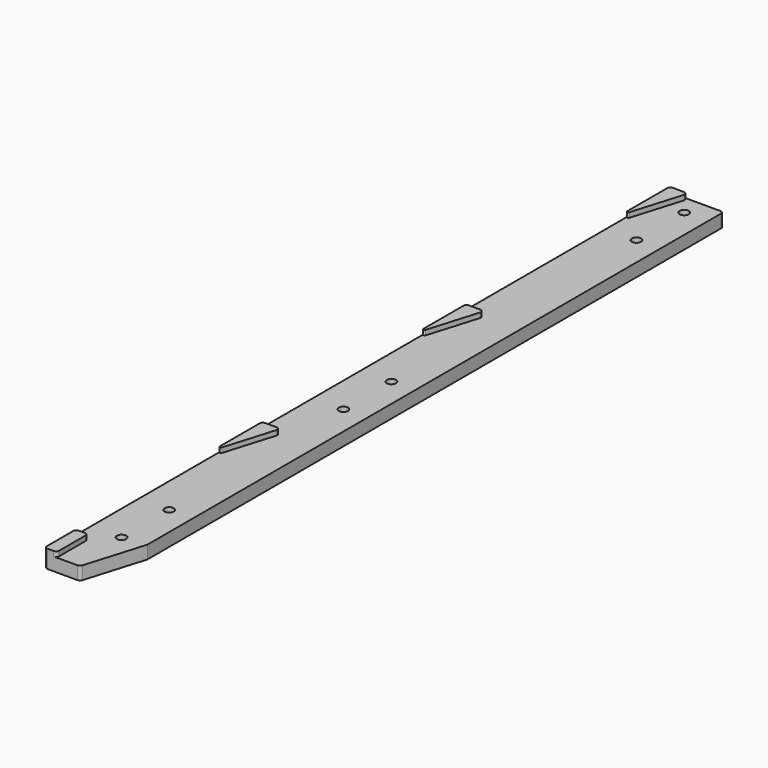
from build123d import *

# Parameters (mm, degrees)
F1_DEPTH = 4.25
F2_W     = 4
F2_H     = 12.7
F3_DEPTH = 1.5875
F4_R     = 1
F5_F1_R  = 0.4
F5_F2_R  = 0.4
F5_F3_R  = 0.4
F7_D     = 3


with BuildPart() as f1:
    # F0 (on Top) → F1 (new body)
    with BuildSketch(Plane.XY):
        Polygon((8.75, 106.9650896668), (-8.75, 106.9650896668), (-8.75, -147.0349103332), (2.75, -147.0349103332), (8.75, -127.0346005735), align=None)
    extrude(amount=-F1_DEPTH)

    # F2 (on face) → F3 (join)
    with BuildSketch(Plane.XY):
        Polygon((-2.75, 24.1850896668), (-8.75, 24.1850896668), (-8.75, 4.1850896668), align=None)
        Polygon((-2.75, -58.5949103332), (-8.75, -58.5949103332), (-8.75, -78.5949103332), align=None)
        with Locations((-6.75, -140.6849103332)):
            Rectangle(F2_W, F2_H)
        Polygon((-2.75, 106.9650896668), (-8.75, 106.9650896668), (-8.75, 86.9650896668), align=None)
    extrude(amount=F3_DEPTH)

    # F4
    f4_edges = [f1.edges().sort_by_distance(p)[0] for p in [
        (-2.75, -58.59491, 0.79375),
        (-8.75, -58.59491, 0.79375),
        (-2.75, 24.18509, 0.79375),
        (-8.75, 24.18509, 0.79375),
        (-2.75, 106.96509, 0.79375),
        (-8.75, 106.96509, -1.33125),
        (8.75, 106.96509, -2.125),
        (-8.75, -147.03491, -1.33125),
        (-4.75, -147.03491, 0.79375),
        (-4.75, -134.33491, 0.79375),
        (-8.75, -134.33491, 0.79375),
        (2.75, -147.03491, -2.125),
    ]]
    fillet(f4_edges, radius=F4_R)

    # F5: fillet of radius 0.4 on 3 edges, made by hand

    # F5_f1
    f5_f1_edges = [f1.edges().sort_by_distance(p)[0] for p in [
        (-8.75, 86.9650896668, 0.79375),
    ]]
    fillet(f5_f1_edges, radius=F5_F1_R)

    # F5_f2
    f5_f2_edges = [f1.edges().sort_by_distance(p)[0] for p in [
        (-8.75, -78.5949103332, 0.79375),
    ]]
    fillet(f5_f2_edges, radius=F5_F2_R)

    # F5_f3
    f5_f3_edges = [f1.edges().sort_by_distance(p)[0] for p in [
        (-8.75, 4.1850896668, 0.79375),
    ]]
    fillet(f5_f3_edges, radius=F5_F3_R)

    # F7 (through all)
    with Locations(Plane.XY):
        with Locations((1.113455, 100.5345896668), (1.113455, 81.1504351225), (1.113455, -18.4210048775), (1.113455, -37.9210048775), (1.113455, -108.6812892063), (1.113455, -128.0654437506)):
            Hole(F7_D / 2)


solid = f1.part
